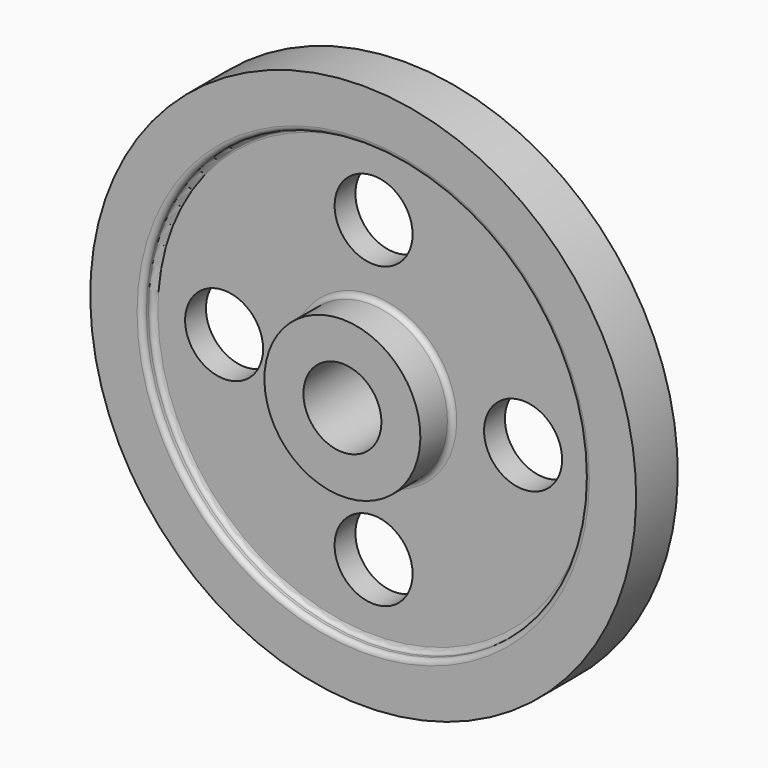
from build123d import *

# Parameters (mm, degrees)
F2_R     = 19.05
F3_DEPTH = 25.4
F4_R     = 2.54


# Not quite as in the source:
# - two fillets or chamfers of one size are made in one step
# - a feature names something its author has since deleted; it is built from what else it names


with BuildPart() as f1:
    # F0 (on Right) → F1 (revolve)
    with BuildSketch(Plane.YZ):
        Polygon((6.35, 38.1), (6.35, 107.95), (12.7, 107.95), (12.7, 133.35), (0, 133.35), (-12.7, 133.35), (-12.7, 107.95), (-6.35, 107.95), (-6.35, 38.1), (0, 38.1), align=None)
        Polygon((25.4, 38.1), (6.35, 38.1), (0, 38.1), (-6.35, 38.1), (-25.4, 38.1), (-25.4, 19.05), (0, 19.05), (25.4, 19.05), align=None)
    revolve(axis=Axis((0, 37.7952009439, 0), (0, 1, 0)))

    # F2 (on face) → F3 (cut)
    with BuildSketch(Plane.XZ.offset(6.35)):
        with Locations((-73.025, 0)):
            Circle(F2_R)
        with Locations((73.025, 0)):
            Circle(F2_R)
        with BuildLine():
            ThreePointArc((19.05, 73.025), (-13.4703841816, 86.4953841816), (0, 53.975))
            ThreePointArc((0, 53.975), (13.4703841816, 59.5546158184), (19.05, 73.025))
        make_face()
        with Locations((0, -73.025)):
            Circle(F2_R)
    extrude(amount=-F3_DEPTH, mode=Mode.SUBTRACT)

    # F4
    f4_edges = [f1.edges().sort_by_distance(p)[0] for p in [
        (0, -6.35, -107.95),
        (0, -12.7, -107.95),
        (0, -6.35, -38.1),
    ]]
    fillet(f4_edges, radius=F4_R)


solid = f1.part
